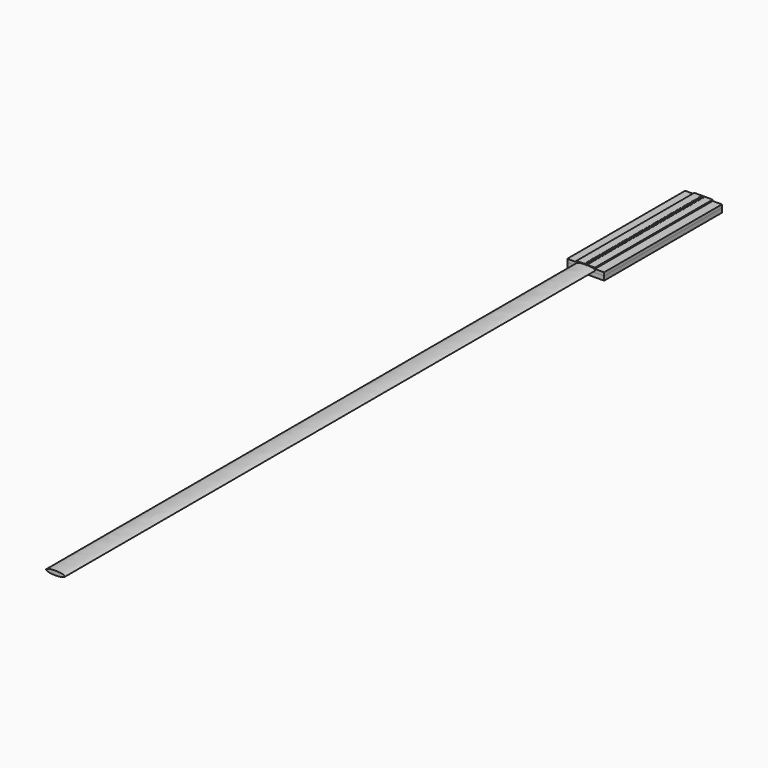
from build123d import *

# Parameters (mm, degrees)
F3_START       = 10
F3_DEPTH       = 90
F1_W           = 1.25
F1_H           = 20
F1_W_2         = 2.5
F7_DEPTH       = 0.44
F8_START       = -0.44
F7_FACE_W      = 5
F7_FACE_H      = 20
F8_DEPTH       = 0.56
F9_W           = 2.5
F9_H           = 20
F10_DEPTH      = 0.06
F11_DEPTH      = 0.1
F12_W          = 0.4
F12_H          = 0.09
F13_DEPTH      = 0.16
F14_DEPTH      = 10
F14_DEPTH_BACK = 10


with BuildPart() as f3:
    # F2 (on Front) → F3 (new body)
    with BuildSketch(Plane.XZ.offset(F3_START)):
        with BuildLine():
            add(Edge.make_bspline(
                [(-1.2761692051, -0.1728112256), (-1.2761692051, -0.6693496106), (0.6380846025, -0.4210804181), (2.5523384102, -0.1728112256), (0.6380846025, 0.0754579668), (-1.2761692051, 0.3237271593), (-1.2761692051, -0.1728112256)],
                knots=[0, 0, 0, 2.0943951024, 2.0943951024, 4.1887902048, 4.1887902048, 6.2831853072, 6.2831853072, 6.2831853072], degree=2, weights=[1, 0.5, 1, 0.5, 1, 0.5, 1]))
        make_face()
    extrude(amount=F3_DEPTH)


with BuildPart() as f7:
    # F1 (on Top) → F7 (new body)
    with BuildSketch(Plane.XY):
        with Locations((-1.875, 0)):
            Rectangle(F1_W, F1_H)
        Rectangle(F1_W_2, F1_H)
        with Locations((1.875, 0)):
            Rectangle(F1_W, F1_H)
    extrude(amount=-F7_DEPTH)

    # F9 (on Top) → F10 (join)
    with BuildSketch(Plane.XY):
        Rectangle(F9_W, F9_H)
    extrude(amount=F10_DEPTH)


with BuildPart() as f8:
    # F7_face (on face) → F8 (new body)
    with BuildSketch(Plane.XY.offset(F8_START)):
        Rectangle(F7_FACE_W, F7_FACE_H)
    extrude(amount=-F8_DEPTH)


with BuildPart() as f11:
    # F11 (new): a face of the model
    f11_faces = [f7.part.faces().sort_by_distance(p)[0] for p in [
        (0, 0, 0.06),
    ]]
    extrude(f11_faces, amount=F11_DEPTH)


with BuildPart() as f13_tool:
    # F12 (on face) → F13 (new body)
    with BuildSketch(Plane.XY.offset(0.16)):
        with Locations((0, -10)):
            Rectangle(F12_W, F12_H)
        with Locations((0, -9.76)):
            Rectangle(F12_W, F12_H)
        with Locations((0, -9.52)):
            Rectangle(F12_W, F12_H)
        with Locations((0, -9.28)):
            Rectangle(F12_W, F12_H)
        with Locations((0, -9.04)):
            Rectangle(F12_W, F12_H)
        with Locations((0, -8.8)):
            Rectangle(F12_W, F12_H)
        with Locations((0, -8.56)):
            Rectangle(F12_W, F12_H)
        with Locations((0, -8.32)):
            Rectangle(F12_W, F12_H)
        with Locations((0, -8.08)):
            Rectangle(F12_W, F12_H)
        with Locations((0, -7.84)):
            Rectangle(F12_W, F12_H)
        with Locations((0, -7.6)):
            Rectangle(F12_W, F12_H)
        with Locations((0, -7.36)):
            Rectangle(F12_W, F12_H)
        with Locations((0, -7.12)):
            Rectangle(F12_W, F12_H)
        with Locations((0, -6.88)):
            Rectangle(F12_W, F12_H)
        with Locations((0, -6.64)):
            Rectangle(F12_W, F12_H)
        with Locations((0, -6.4)):
            Rectangle(F12_W, F12_H)
        with Locations((0, -6.16)):
            Rectangle(F12_W, F12_H)
        with Locations((0, -5.92)):
            Rectangle(F12_W, F12_H)
        with Locations((0, -5.68)):
            Rectangle(F12_W, F12_H)
        with Locations((0, -5.44)):
            Rectangle(F12_W, F12_H)
        with Locations((0, -5.2)):
            Rectangle(F12_W, F12_H)
        with Locations((0, -4.96)):
            Rectangle(F12_W, F12_H)
        with Locations((0, -4.72)):
            Rectangle(F12_W, F12_H)
        with Locations((0, -4.48)):
            Rectangle(F12_W, F12_H)
        with Locations((0, -4.24)):
            Rectangle(F12_W, F12_H)
        with Locations((0, -4)):
            Rectangle(F12_W, F12_H)
        with Locations((0, -3.76)):
            Rectangle(F12_W, F12_H)
        with Locations((0, -3.52)):
            Rectangle(F12_W, F12_H)
        with Locations((0, -3.28)):
            Rectangle(F12_W, F12_H)
        with Locations((0, -3.04)):
            Rectangle(F12_W, F12_H)
        with Locations((0, -2.8)):
            Rectangle(F12_W, F12_H)
        with Locations((0, -2.56)):
            Rectangle(F12_W, F12_H)
        with Locations((0, -2.32)):
            Rectangle(F12_W, F12_H)
        with Locations((0, -2.08)):
            Rectangle(F12_W, F12_H)
        with Locations((0, -1.84)):
            Rectangle(F12_W, F12_H)
        with Locations((0, -1.6)):
            Rectangle(F12_W, F12_H)
        with Locations((0, -1.36)):
            Rectangle(F12_W, F12_H)
        with Locations((0, -1.12)):
            Rectangle(F12_W, F12_H)
        with Locations((0, -0.88)):
            Rectangle(F12_W, F12_H)
        with Locations((0, -0.64)):
            Rectangle(F12_W, F12_H)
        with Locations((0, -0.4)):
            Rectangle(F12_W, F12_H)
        with Locations((0, -0.16)):
            Rectangle(F12_W, F12_H)
        with Locations((0, 0.08)):
            Rectangle(F12_W, F12_H)
        with Locations((0, 0.32)):
            Rectangle(F12_W, F12_H)
        with Locations((0, 0.56)):
            Rectangle(F12_W, F12_H)
        with Locations((0, 0.8)):
            Rectangle(F12_W, F12_H)
        with Locations((0, 1.04)):
            Rectangle(F12_W, F12_H)
        with Locations((0, 1.28)):
            Rectangle(F12_W, F12_H)
        with Locations((0, 1.52)):
            Rectangle(F12_W, F12_H)
        with Locations((0, 1.76)):
            Rectangle(F12_W, F12_H)
        with Locations((0, 2)):
            Rectangle(F12_W, F12_H)
        with Locations((0, 2.24)):
            Rectangle(F12_W, F12_H)
        with Locations((0, 2.48)):
            Rectangle(F12_W, F12_H)
        with Locations((0, 2.72)):
            Rectangle(F12_W, F12_H)
        with Locations((0, 2.96)):
            Rectangle(F12_W, F12_H)
        with Locations((0, 3.2)):
            Rectangle(F12_W, F12_H)
        with Locations((0, 3.44)):
            Rectangle(F12_W, F12_H)
        with Locations((0, 3.68)):
            Rectangle(F12_W, F12_H)
        with Locations((0, 3.92)):
            Rectangle(F12_W, F12_H)
        with Locations((0, 4.16)):
            Rectangle(F12_W, F12_H)
        with Locations((0, 4.4)):
            Rectangle(F12_W, F12_H)
        with Locations((0, 4.64)):
            Rectangle(F12_W, F12_H)
        with Locations((0, 4.88)):
            Rectangle(F12_W, F12_H)
        with Locations((0, 5.12)):
            Rectangle(F12_W, F12_H)
        with Locations((0, 5.36)):
            Rectangle(F12_W, F12_H)
        with Locations((0, 5.6)):
            Rectangle(F12_W, F12_H)
        with Locations((0, 5.84)):
            Rectangle(F12_W, F12_H)
        with Locations((0, 6.08)):
            Rectangle(F12_W, F12_H)
        with Locations((0, 6.32)):
            Rectangle(F12_W, F12_H)
        with Locations((0, 6.56)):
            Rectangle(F12_W, F12_H)
        with Locations((0, 6.8)):
            Rectangle(F12_W, F12_H)
        with Locations((0, 7.04)):
            Rectangle(F12_W, F12_H)
        with Locations((0, 7.28)):
            Rectangle(F12_W, F12_H)
        with Locations((0, 7.52)):
            Rectangle(F12_W, F12_H)
        with Locations((0, 7.76)):
            Rectangle(F12_W, F12_H)
        with Locations((0, 8)):
            Rectangle(F12_W, F12_H)
        with Locations((0, 8.24)):
            Rectangle(F12_W, F12_H)
        with Locations((0, 8.48)):
            Rectangle(F12_W, F12_H)
        with Locations((0, 8.72)):
            Rectangle(F12_W, F12_H)
        with Locations((0, 8.96)):
            Rectangle(F12_W, F12_H)
        with Locations((0, 9.2)):
            Rectangle(F12_W, F12_H)
        with Locations((0, 9.44)):
            Rectangle(F12_W, F12_H)
        with Locations((0, 9.68)):
            Rectangle(F12_W, F12_H)
        with Locations((0, 9.92)):
            Rectangle(F12_W, F12_H)
        with Locations((0, 10.16)):
            Rectangle(F12_W, F12_H)
        with Locations((0, 10.4)):
            Rectangle(F12_W, F12_H)
        with Locations((0, 10.64)):
            Rectangle(F12_W, F12_H)
        with Locations((0, 10.88)):
            Rectangle(F12_W, F12_H)
        with Locations((0, 11.12)):
            Rectangle(F12_W, F12_H)
        with Locations((0, 11.36)):
            Rectangle(F12_W, F12_H)
        with Locations((0, 11.6)):
            Rectangle(F12_W, F12_H)
        with Locations((0, 11.84)):
            Rectangle(F12_W, F12_H)
        with Locations((0, 12.08)):
            Rectangle(F12_W, F12_H)
        with Locations((0, 12.32)):
            Rectangle(F12_W, F12_H)
        with Locations((0, 12.56)):
            Rectangle(F12_W, F12_H)
        with Locations((0, 12.8)):
            Rectangle(F12_W, F12_H)
        with Locations((0, 13.04)):
            Rectangle(F12_W, F12_H)
        with Locations((0, 13.28)):
            Rectangle(F12_W, F12_H)
        with Locations((0, 13.52)):
            Rectangle(F12_W, F12_H)
        with Locations((0, 13.76)):
            Rectangle(F12_W, F12_H)
    extrude(amount=-F13_DEPTH)


with BuildPart() as f3_1:
    add(f3.part)

    # F13: cut by f13_tool
    add(f13_tool.part, mode=Mode.SUBTRACT)


with BuildPart() as f7_1:
    add(f7.part)

    # F13: cut by f13_tool
    add(f13_tool.part, mode=Mode.SUBTRACT)


with BuildPart() as f11_1:
    add(f11.part)

    # F13: cut by f13_tool
    add(f13_tool.part, mode=Mode.SUBTRACT)


with BuildPart() as f14:
    # F2 (on Front) → F14 (new body, two sides)
    with BuildSketch(Plane.XZ) as f14_sk:
        with BuildLine():
            add(Edge.make_bspline(
                [(-1.2761692051, -0.1728112256), (-1.2761692051, -0.6693496106), (0.6380846025, -0.4210804181), (2.5523384102, -0.1728112256), (0.6380846025, 0.0754579668), (-1.2761692051, 0.3237271593), (-1.2761692051, -0.1728112256)],
                knots=[0, 0, 0, 2.0943951024, 2.0943951024, 4.1887902048, 4.1887902048, 6.2831853072, 6.2831853072, 6.2831853072], degree=2, weights=[1, 0.5, 1, 0.5, 1, 0.5, 1]))
        make_face()
    extrude(amount=F14_DEPTH)
    extrude(f14_sk.sketch, amount=-F14_DEPTH_BACK)


solid = Compound([f8.part, f3_1.part, f7_1.part, f11_1.part, f14.part])
